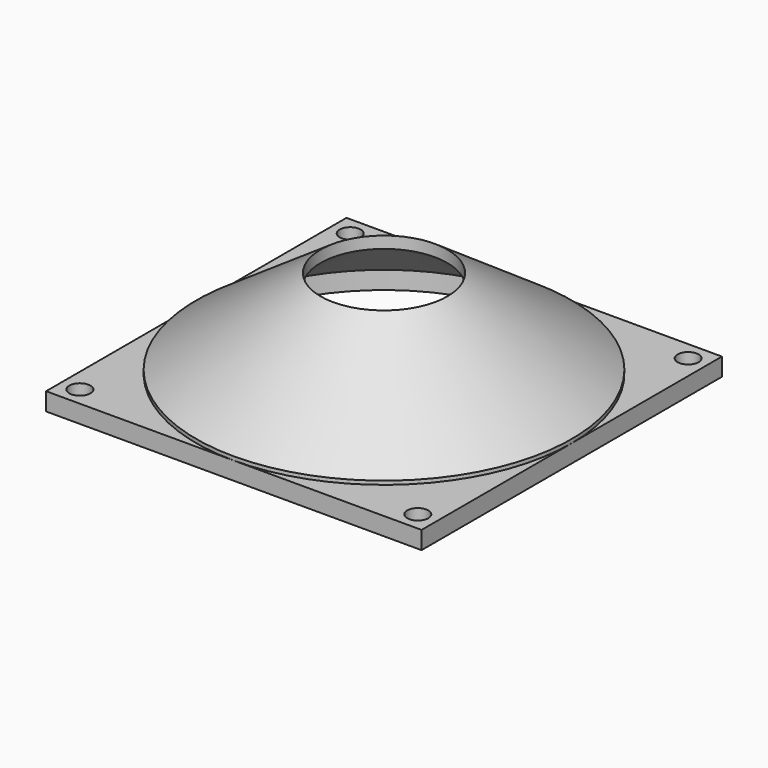
from build123d import *

# Parameters (mm, degrees)
F0_W     = 80
F0_H     = 80
F0_R     = 2.25
F0_R_2   = 37.5
F1_DEPTH = 3.8


# Not quite as in the source:
# - a feature names something its author has since deleted; it is built from what else it names


with BuildPart() as f1:
    # F0 (on Top) → F1 (new body)
    with BuildSketch(Plane.XY):
        Rectangle(F0_W, F0_H)
        with Locations((-36, -36)):
            Circle(F0_R, mode=Mode.SUBTRACT)
        with Locations((36, -36)):
            Circle(F0_R, mode=Mode.SUBTRACT)
        with Locations((-36, 36)):
            Circle(F0_R, mode=Mode.SUBTRACT)
        Circle(F0_R_2, mode=Mode.SUBTRACT)
        with Locations((36, 36)):
            Circle(F0_R, mode=Mode.SUBTRACT)
    extrude(amount=F1_DEPTH)

    # F2 (on Right) → F3 (revolve)
    with BuildSketch(Plane.YZ):
        Polygon((-40, 0), (-37.5, 0), (-37.5, 3.8), (-13.5, 20.2198829502), (-13.5, 22.7198829502), (-40, 4.589595526), (-40, 3.8), align=None)
    revolve(axis=Axis((0, 0, 27.8761722147), (0, 0, 1)))


solid = f1.part
